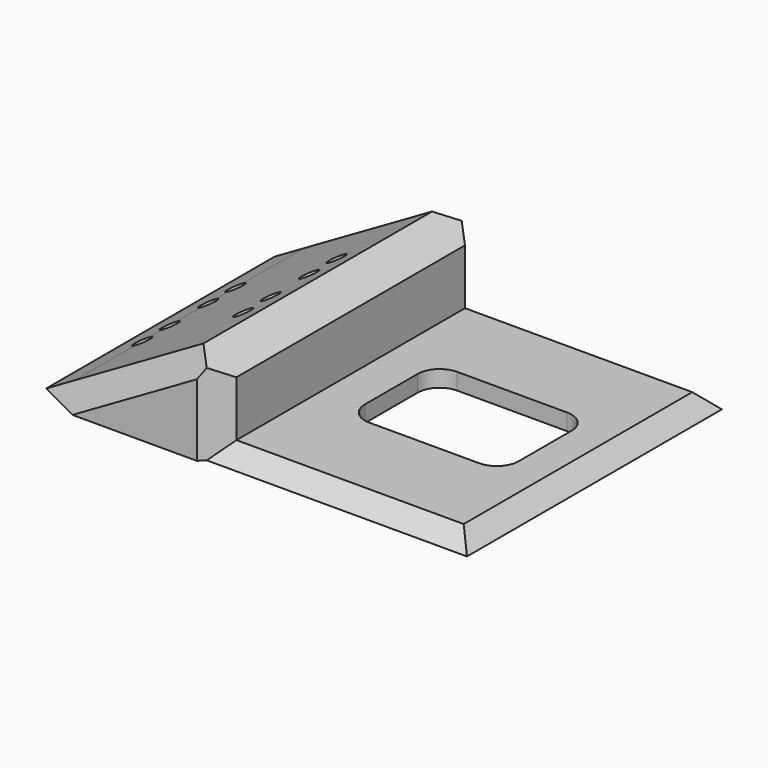
from build123d import *

# Parameters (mm, degrees)
F0_W          = 101.6
F0_H          = 76.2
F2_DEPTH      = 3.81
F3_DEPTH      = 38.1
F3_DEPTH_BACK = 38.1
F5_DEPTH      = 101.6
F6_R          = 2.032
F7_DEPTH      = 25.4
F9_R          = 3.175
F9_R_2        = 2.032
F10_DEPTH     = 25.4
F11_W         = 35.56
F11_H         = 25.4
F12_DEPTH     = 25.4
F13_T1_DEPTH  = 102.3282991577
F13_T3_DEPTH  = 70.6700590666
F13_T5_DEPTH  = 34.6541495789
F13_T11_DEPTH = 70.6700590666
F13_T16_DEPTH = 47.7182991577
F14_SIZE      = 5.08
F15_T1_DEPTH  = 71.0624204228
F15_T3_DEPTH  = 110.5507880402
F15_T5_DEPTH  = 71.0624204227
F16_R         = 5.08


# Not quite as in the source:
# - a fillet or chamfer that OpenCascade refuses, or shapes differently, is made with other operations: its cross-section is extruded or revolved along the edge and cut away or added


with BuildPart() as f2:
    # F0 (on Top) → F2 (new body)
    with BuildSketch(Plane.XY):
        with Locations((-38.1367237687, 0)):
            Rectangle(F0_W, F0_H)
    extrude(amount=F2_DEPTH)

    # F1 (on Front) → F3 (join, two sides)
    with BuildSketch(Plane.XZ) as f3_sk:
        Polygon((-44.9426332565, 25.4), (-88.9367237687, 0), (-44.9426332565, 0), align=None)
    extrude(amount=F3_DEPTH)
    extrude(f3_sk.sketch, amount=-F3_DEPTH_BACK)

    # F4 (on face) → F5 (cut)
    with BuildSketch(Plane.XZ.offset(38.1)):
        Polygon((-88.9367237687, 0), (-82.3376101919, 3.81), (-88.9367237687, 3.81), align=None)
    extrude(amount=-F5_DEPTH, mode=Mode.SUBTRACT)

    # F6 (on face) → F7 (cut)
    with BuildSketch(Plane(origin=(-22.2341809422, 0, 38.5107310565), x_dir=(0.8660254038, 0, 0.5), z_dir=(-0.5, 0, 0.8660254038))):
        with Locations((-69.4014621131, -13.4874)):
            Circle(F6_R)
        with Locations((-69.4014621131, -5.588)):
            Circle(F6_R)
        with Locations((-69.4014621131, 5.5626)):
            Circle(F6_R)
        with Locations((-69.4014621131, 13.462)):
            Circle(F6_R)
        with Locations((-42.4520621131, 13.462)):
            Circle(F6_R)
        with Locations((-42.4520621131, -5.588)):
            Circle(F6_R)
        with Locations((-42.4520621131, -13.4874)):
            Circle(F6_R)
        with Locations((-42.4520621131, 5.5626)):
            Circle(F6_R)
    extrude(amount=-F7_DEPTH, mode=Mode.SUBTRACT)

    # F9 (on offset) → F10 (cut)
    with BuildSketch(Plane(origin=(-20.3291809422, 0, 35.2111742681), x_dir=(0.8660254038, 0, 0.5), z_dir=(-0.5, 0, 0.8660254038))):
        with Locations((-69.4014621131, 13.462)):
            Circle(F9_R)
        with Locations((-69.4014621131, 13.462)):
            Circle(F9_R_2, mode=Mode.SUBTRACT)
        with Locations((-69.4014621131, 5.5626)):
            Circle(F9_R)
        with Locations((-69.4014621131, 5.5626)):
            Circle(F9_R_2, mode=Mode.SUBTRACT)
        with Locations((-69.4014621131, -5.588)):
            Circle(F9_R)
        with Locations((-69.4014621131, -5.588)):
            Circle(F9_R_2, mode=Mode.SUBTRACT)
        with Locations((-69.4014621131, -13.4874)):
            Circle(F9_R)
        with Locations((-69.4014621131, -13.4874)):
            Circle(F9_R_2, mode=Mode.SUBTRACT)
        with Locations((-42.4520621131, -5.588)):
            Circle(F9_R)
        with Locations((-42.4520621131, -5.588)):
            Circle(F9_R_2, mode=Mode.SUBTRACT)
        with Locations((-42.4520621131, -13.4874)):
            Circle(F9_R)
        with Locations((-42.4520621131, -13.4874)):
            Circle(F9_R_2, mode=Mode.SUBTRACT)
        with Locations((-42.4520621131, 5.5626)):
            Circle(F9_R)
        with Locations((-42.4520621131, 5.5626)):
            Circle(F9_R_2, mode=Mode.SUBTRACT)
        with Locations((-42.4520621131, 13.462)):
            Circle(F9_R)
        with Locations((-42.4520621131, 13.462)):
            Circle(F9_R_2, mode=Mode.SUBTRACT)
    extrude(amount=-F10_DEPTH, mode=Mode.SUBTRACT)

    # F11 (on face) → F12 (cut)
    with BuildSketch(Plane(origin=(0, 0, 0), x_dir=(1, 0, 0), z_dir=(0, 0, -1))):
        with Locations((-17.78, 0)):
            Rectangle(F11_W, F11_H)
    extrude(amount=-F12_DEPTH, mode=Mode.SUBTRACT)

    # F13: chamfer of 5.08 on 4 edges, made by hand

    # F13_s2 → F13_t1 (cut)
    with BuildSketch(Plane.XZ.offset(-51.1641495789)):
        Polygon((12.6632762313, -1.27), (7.5832762313, 3.81), (12.6632762313, 3.81), align=None)
    extrude(amount=F13_T1_DEPTH, mode=Mode.SUBTRACT)

    # F13_s4 → F13_t3 (cut)
    with BuildSketch(Plane.YZ.offset(-44.9426332565)):
        Polygon((-38.1, -1.27), (-33.02, 3.81), (-38.1, 3.81), align=None)
        Polygon((38.1, -1.27), (33.02, 3.81), (38.1, 3.81), align=None)
    extrude(amount=F13_T3_DEPTH, mode=Mode.SUBTRACT)

    # F13_s6 → F13_t5 (cut)
    with BuildSketch(Plane.XY.offset(3.81)):
        Polygon((-50.0226332565, 38.1), (-44.9426332565, 33.02), (-44.9426332565, 38.1), align=None)
    extrude(amount=F13_T5_DEPTH, mode=Mode.SUBTRACT)


with BuildPart() as f13_tool9:
    # F13_s10 → F13_t11 (new body)
    with BuildSketch(Plane.YZ.offset(12.6632762313)):
        Polygon((38.1, -1.27), (33.02, 3.81), (38.1, 3.81), align=None)
    extrude(amount=-F13_T11_DEPTH)

    split(bisect_by=Plane.XY, keep=Keep.TOP)

    split(bisect_by=Plane.YZ.offset(-44.9426332565), keep=Keep.BOTTOM)


with BuildPart() as f13_tool14:
    # F13_s15 → F13_t16 (new body)
    with BuildSketch(Plane.XY.offset(-9.2541495789)):
        Polygon((-50.0226332565, 38.1), (-44.9426332565, 33.02), (-44.9426332565, 38.1), align=None)
    extrude(amount=F13_T16_DEPTH)

    split(bisect_by=Plane.XY, keep=Keep.TOP)

    split(bisect_by=Plane.XY.offset(3.81), keep=Keep.BOTTOM)


with BuildPart() as f13_tool9_1:
    add(f13_tool9.part)

    # F13_t19: intersect F13_tool14
    add(f13_tool14.part, mode=Mode.INTERSECT)


with BuildPart() as f2_1:
    add(f2.part)

    # F13_t7: cut F13_tool9
    add(f13_tool9_1.part, mode=Mode.SUBTRACT)

    # F14
    f14_edges = [f2_1.edges().sort_by_distance(p)[0] for p in [
        (-44.942633, -38.1, 12.7),
    ]]
    chamfer(f14_edges, length=F14_SIZE)

    # F15: chamfer of 5.08 on 3 edges, made by hand

    # F15_s2 → F15_t1 (cut)
    with BuildSketch(Plane(origin=(-16.4745669001, 0, -9.5115956346), x_dir=(0, 1, 0), z_dir=(-0.8660254038, 0, -0.5))):
        Polygon((-38.1, -39.3883618844), (-33.02, -44.4683618844), (-38.1, -44.4683618844), align=None)
    extrude(amount=F15_T1_DEPTH, mode=Mode.SUBTRACT)

    # F15_s4 → F15_t3 (cut)
    with BuildSketch(Plane.XZ.offset(-55.2753940201)):
        Polygon((-52.5626332565, 21.0005909488), (-44.9426332565, 16.6011818976), (-44.9426332565, 25.4), align=None)
    extrude(amount=F15_T3_DEPTH, mode=Mode.SUBTRACT)

    # F15_s6 → F15_t5 (cut)
    with BuildSketch(Plane(origin=(-78.0164282407, 0, -45.042805846), x_dir=(0, 1, 0), z_dir=(0.8660254038, 0, 0.5))):
        Polygon((33.02, 44.4683618844), (38.1, 39.3883618844), (38.1, 44.4683618844), align=None)
    extrude(amount=F15_T5_DEPTH, mode=Mode.SUBTRACT)

    # F16
    f16_edges = [f2_1.edges().sort_by_distance(p)[0] for p in [
        (-35.56, -12.7, 1.905),
        (-35.56, 12.7, 1.905),
        (0, 12.7, 1.905),
        (0, -12.7, 1.905),
    ]]
    fillet(f16_edges, radius=F16_R)


solid = f2_1.part
